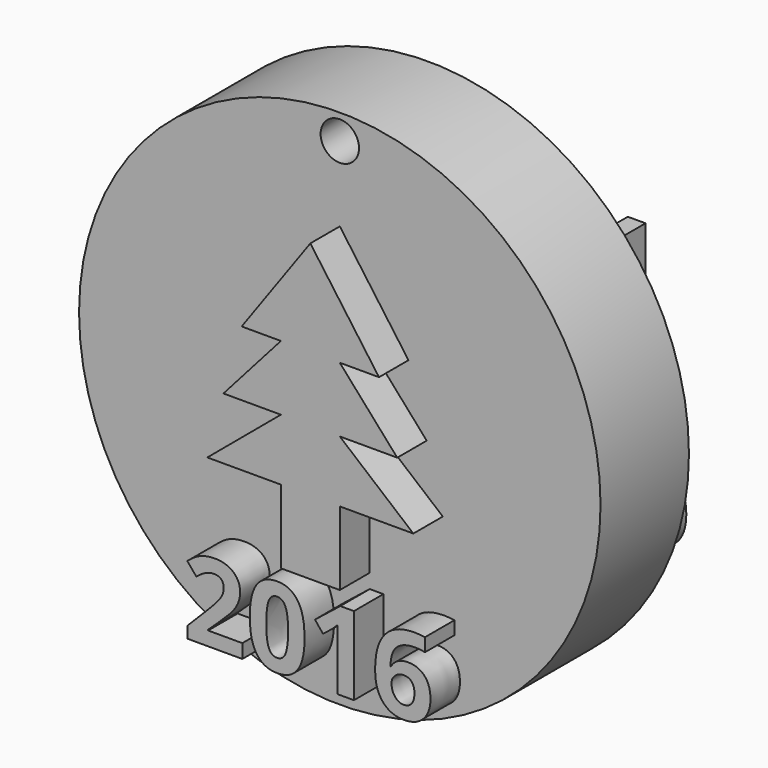
from build123d import *

# Parameters (mm, degrees)
F2_DEPTH       = 25.4
F0_R           = 44.9578799501
F3_DEPTH       = 19.05
F4_R           = 3.3092768992
F5_DEPTH       = 80.01
F6_TEXT_SIZE   = 18.9437832462
F7_DEPTH       = 6.35
F8_TEXT_SIZE   = 24.4254461361
F8_TEXT_SIZE_2 = 17.0645019457
F9_DEPTH       = 6.35


# Not quite as in the source:
# - Text() gives the source's letters only with a copy of the font that has no kerning and outlines rounded to 1/6400 em; it was checked with that copy


with BuildPart() as f2:
    # F1 (on face) → F2 (new body)
    with BuildSketch(Plane.XZ):
        Polygon((-5.08, -23.3135717287), (0, -23.3135717287), (5.08, -23.3135717287), (5.08, -10.6135717287), (17.7594460547, -10.6135717287), (5.08, 0), (14.9845322594, 0), (5.08, 11.192150414), (11.8396300822, 11.192150414), (0, 27.6566352695), (-11.8396300822, 11.192150414), (-5.08, 11.192150414), (-14.9845322594, 0), (-5.08, 0), (-17.7594460547, -10.6135717287), (-5.08, -10.6135717287), align=None)
    extrude(amount=F2_DEPTH)

    # F0 (on Front) → F3 (join)
    with BuildSketch(Plane.XZ):
        Circle(F0_R)
    extrude(amount=F3_DEPTH)

    # F4 (on face) → F5 (cut)
    with BuildSketch(Plane.XZ.offset(19.05)):
        with Locations((0, 40.6062342227)):
            Circle(F4_R)
    extrude(amount=-F5_DEPTH, mode=Mode.SUBTRACT)

    # F6 (on face) → F7 (join)
    with BuildSketch(Plane.XZ.offset(19.05)):
        with Locations((-21.939268972, -39.2412977178)):
            Text('2016', F6_TEXT_SIZE, font='Open Sans', font_style=FontStyle.BOLD, text_align=(TextAlign.LEFT, TextAlign.BOTTOM))
    extrude(amount=F7_DEPTH)

    # F8 (on face) → F9 (join)
    with BuildSketch(Plane(origin=(0, 0, 0), x_dir=(-1, 0, 0), z_dir=(0, 1, 0))):
        with Locations((-34.7852701262, 10.8951807061)):
            Text('Merry', F8_TEXT_SIZE, font='Open Sans', text_align=(TextAlign.LEFT, TextAlign.BOTTOM))
        with Locations((-40.463531549, -19.593712874)):
            Text('Christmas', F8_TEXT_SIZE_2, font='Open Sans', text_align=(TextAlign.LEFT, TextAlign.BOTTOM))
    extrude(amount=F9_DEPTH)


solid = f2.part
